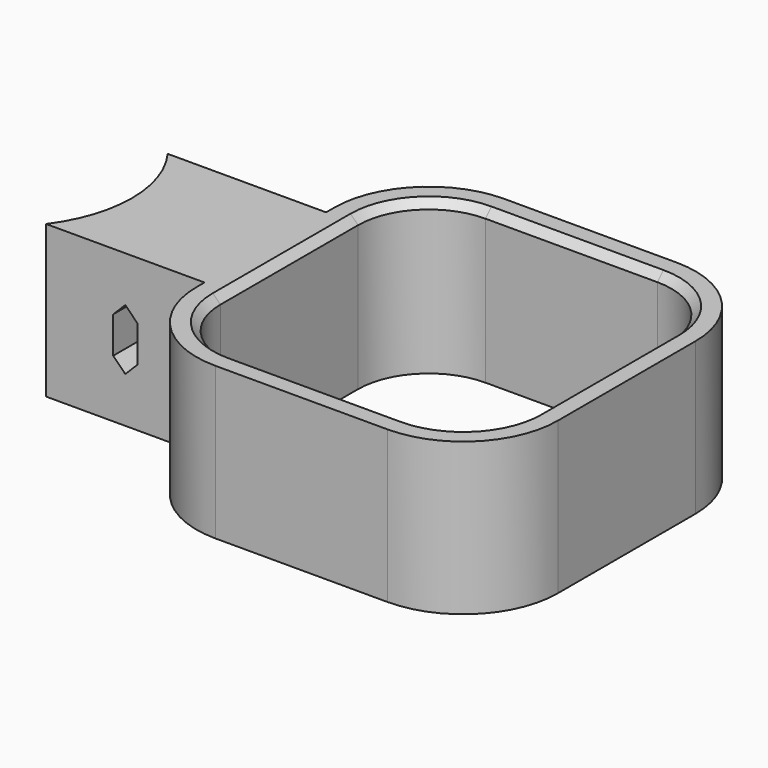
from build123d import *

# Parameters (mm, degrees)
F0_W     = 2
F0_H     = 12.7
F1_DEPTH = 12.7
F2_SIZE  = 0.635
F3_W     = 2.032
F3_H     = 5.08
F4_DEPTH = 25.4
F5_SIZE  = 1.01599


# Not quite as in the source:
# - a fillet or chamfer is up to 0.001 mm smaller than in the source, because OpenCascade refuses the exact size


with BuildPart() as f1:
    # F0 (on Top) → F1 (new body)
    with BuildSketch(Plane.XY):
        with BuildLine():
            Line((-15.1, -6.35), (-15.1, 6.35))
            Line((-15.1, 6.35), (-28.34, 6.35))
            ThreePointArc((-28.34, 6.35), (-26.7817380481, 3.3434490418), (-26.2442648116, 0))
            ThreePointArc((-26.2442648116, 0), (-26.7817380481, -3.3434490418), (-28.34, -6.35))
            Line((-28.34, -6.35), (-15.1, -6.35))
        make_face()
        with Locations((-14.1, 0)):
            Rectangle(F0_W, F0_H)
        with BuildLine():
            ThreePointArc((7.19, 13.1), (11.3690010768, 11.3690010768), (13.1, 7.19))
            Line((13.1, 7.19), (13.1, -7.19))
            ThreePointArc((13.1, -7.19), (11.3690010768, -11.3690010768), (7.19, -13.1))
            Line((7.19, -13.1), (-7.19, -13.1))
            ThreePointArc((-7.19, -13.1), (-11.3690010768, -11.3690010768), (-13.1, -7.19))
            Line((-13.1, -7.19), (-13.1, -6.35))
            Line((-13.1, -6.35), (-15.1, -6.35))
            Line((-15.1, -6.35), (-15.1, -7.19))
            ThreePointArc((-15.1, -7.19), (-12.7832146392, -12.7832146392), (-7.19, -15.1))
            Line((-7.19, -15.1), (7.19, -15.1))
            ThreePointArc((7.19, -15.1), (12.7832146392, -12.7832146392), (15.1, -7.19))
            Line((15.1, -7.19), (15.1, 7.19))
            ThreePointArc((15.1, 7.19), (12.7832146392, 12.7832146392), (7.19, 15.1))
            Line((7.19, 15.1), (-7.19, 15.1))
            ThreePointArc((-7.19, 15.1), (-12.7832146392, 12.7832146392), (-15.1, 7.19))
            Line((-15.1, 7.19), (-15.1, 6.35))
            Line((-15.1, 6.35), (-13.1, 6.35))
            Line((-13.1, 6.35), (-13.1, 7.19))
            ThreePointArc((-13.1, 7.19), (-11.3690010768, 11.3690010768), (-7.19, 13.1))
            Line((-7.19, 13.1), (7.19, 13.1))
        make_face()
    extrude(amount=F1_DEPTH)

    # F2
    f2_edges = [f1.edges().sort_by_distance(p)[0] for p in [
        (-11.369001, 11.369001, 12.7),
        (0, 13.1, 12.7),
        (11.369001, 11.369001, 12.7),
        (13.1, 0, 12.7),
        (11.369001, -11.369001, 12.7),
        (0, -13.1, 12.7),
        (-11.369001, -11.369001, 12.7),
        (-13.1, 0, 12.7),
    ]]
    chamfer(f2_edges, length=F2_SIZE)

    # F3 (on face) → F4 (cut)
    with BuildSketch(Plane.XZ.offset(6.35)):
        with Locations((-21.72, 6.35)):
            Rectangle(F3_W, F3_H)
    extrude(amount=-F4_DEPTH, mode=Mode.SUBTRACT)

    # F5 (size 1.016 in the source; OpenCascade refuses exactly that, so slightly less here)
    f5_edges = [f1.edges().sort_by_distance(p)[0] for p in [
        (-22.736, 0, 3.81),
        (-20.704, 0, 3.81),
        (-20.704, 0, 8.89),
        (-22.736, 0, 8.89),
    ]]
    chamfer(f5_edges, length=F5_SIZE)


solid = f1.part
